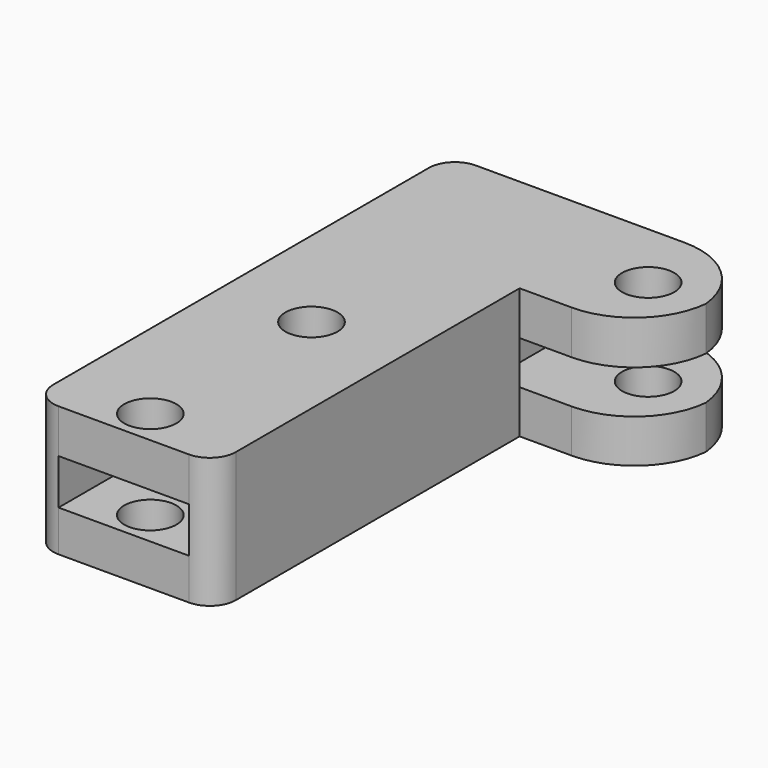
from build123d import *

# Parameters (mm, degrees)
F0_R            = 1.27
F1_DEPTH        = 6.35
F3_W            = 6.858
F3_H            = 2.1082
F4_DEPTH        = 7.62
F5_R            = 1.27
F6_W            = 6.35
F6_H            = 2.2097155452
F7_DEPTH        = 6.35
F9_D            = 2.54
F9_CBORE_D      = 2.54
F9_CBORE_DEPTH  = 6.35
F11_D           = 2.54
F11_CBORE_D     = 2.54
F11_CBORE_DEPTH = 6.35
F12_T1_DEPTH    = 21.1836
F12_T3_DEPTH    = 21.1582


# Not quite as in the source:
# - a fillet or chamfer that OpenCascade refuses, or shapes differently, is made with other operations: its cross-section is extruded or revolved along the edge and cut away or added


with BuildPart() as f1:
    # F0 (on Top) → F1 (new body)
    with BuildSketch(Plane.XY):
        Polygon((6.35, 0), (0, 0), (-8.89, 0), (-8.89, -6.858), (-8.89, -25.4), (0, -25.4), (0, -6.858), (6.35, -6.858), align=None)
        with Locations((3.5186004825, -3.429)):
            Circle(F0_R, mode=Mode.SUBTRACT)
    extrude(amount=F1_DEPTH)

    # F3 (on face) → F4 (cut)
    with BuildSketch(Plane.YZ.offset(6.35)):
        with Locations((-3.429, 3.1623)):
            Rectangle(F3_W, F3_H)
    extrude(amount=-F4_DEPTH, mode=Mode.SUBTRACT)

    # F5
    f5_edges = [f1.edges().sort_by_distance(p)[0] for p in [
        (0, -25.4, 3.175),
        (-8.89, -25.4, 3.175),
        (-8.89, 0, 3.175),
    ]]
    fillet(f5_edges, radius=F5_R)

    # F6 (on face) → F7 (cut)
    with BuildSketch(Plane.XZ.offset(25.4)):
        with Locations((-4.445, 3.1112665311)):
            Rectangle(F6_W, F6_H)
    extrude(amount=-F7_DEPTH, mode=Mode.SUBTRACT)

    # F9 (through all)
    with Locations(Plane.XY.offset(6.35)):
        with Locations((-4.5120492578, -23.6996337771)):
            CounterBoreHole(F9_D / 2, F9_CBORE_D / 2, F9_CBORE_DEPTH)

    # F11 (through all)
    with Locations(Plane.XY.offset(6.35)):
        with Locations((-4.445, -13.97)):
            CounterBoreHole(F11_D / 2, F11_CBORE_D / 2, F11_CBORE_DEPTH)

    # F12: fillet of radius 3.81 on 4 edges, made by hand

    # F12_s2 → F12_t1 (cut)
    with BuildSketch(Plane.XY.offset(-5.3086)):
        with BuildLine():
            ThreePointArc((6.35, -3.048), (5.2340768363, -5.7420768363), (2.54, -6.858))
            Line((2.54, -6.858), (6.35, -6.858))
            Line((6.35, -6.858), (6.35, -3.048))
        make_face()
        with BuildLine():
            ThreePointArc((2.54, 0), (5.2340768363, -1.1159231637), (6.35, -3.81))
            Line((6.35, -3.81), (6.35, 0))
            Line((6.35, 0), (2.54, 0))
        make_face()
    extrude(amount=F12_T1_DEPTH, mode=Mode.SUBTRACT)

    # F12_s4 → F12_t3 (cut)
    with BuildSketch(Plane.XY.offset(-9.525)):
        with BuildLine():
            ThreePointArc((6.35, -3.048), (5.2340768363, -5.7420768363), (2.54, -6.858))
            Line((2.54, -6.858), (6.35, -6.858))
            Line((6.35, -6.858), (6.35, -3.048))
        make_face()
        with BuildLine():
            ThreePointArc((2.54, 0), (5.2340768363, -1.1159231637), (6.35, -3.81))
            Line((6.35, -3.81), (6.35, 0))
            Line((6.35, 0), (2.54, 0))
        make_face()
    extrude(amount=F12_T3_DEPTH, mode=Mode.SUBTRACT)


solid = f1.part
